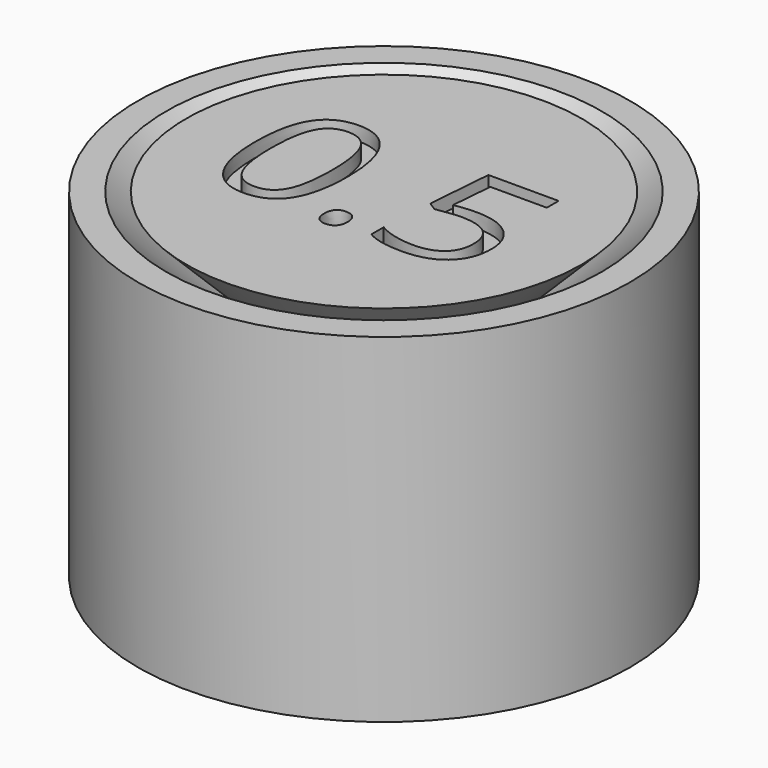
from build123d import *

# Parameters (mm, degrees)
F2_TEXT_SIZE = 6.9979267816
F3_DEPTH     = 0.5
F4_W         = 7
F4_H         = 1.5
F5_DEPTH     = 3


# Not quite as in the source:
# - Text() gives the source's letters only with a copy of the font that has no kerning and outlines rounded to 1/6400 em; it was checked with that copy


with BuildPart() as f1:
    # F0 (on Front) → F1 (revolve)
    with BuildSketch(Plane.XZ):
        Polygon((0, 12), (0, 0), (7, 0), (2, 5), (2, 7), (7, 12), align=None)
    revolve(axis=Axis((0, 0, 6), (0, 0, -1)))

    # F2 (on face) → F3 (cut)
    with BuildSketch(Plane.XY.offset(12)):
        with Locations((-4.9894163385, -2.4183529895)):
            Text('0.5', F2_TEXT_SIZE, font='Open Sans', text_align=(TextAlign.LEFT, TextAlign.BOTTOM))
    extrude(amount=-F3_DEPTH, mode=Mode.SUBTRACT)

    # F4 (on face) → F5 (cut)
    with BuildSketch(Plane(origin=(0, 0, 0), x_dir=(1, 0, 0), z_dir=(0, 0, -1))):
        Rectangle(F4_W, F4_H)
    extrude(amount=-F5_DEPTH, mode=Mode.SUBTRACT)


with BuildPart() as f1b:
    # F0 (on Front) → F1, piece 2 (revolve)
    with BuildSketch(Plane.XZ):
        Polygon((2.5, 5.2071067812), (7.7071067812, 0), (8.7071067812, 0), (8.7071067812, 12), (7.7071067812, 12), (2.5, 6.7928932188), align=None)
    revolve(axis=Axis((0, 0, 6), (0, 0, -1)))


solid = Compound([f1.part, f1b.part])
